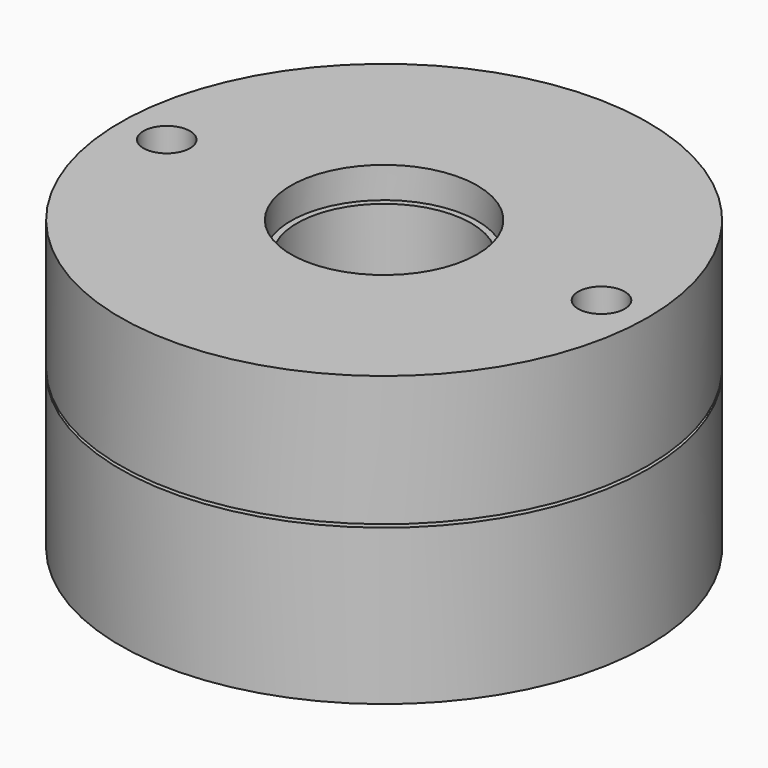
from build123d import *

# Parameters (mm, degrees)
F5_R      = 17
F5_W      = 21.2132034356
F5_H      = 21.2132034356
F5_R_2    = 8.1
F5_R_3    = 6
F6_DEPTH  = 0.5
F7_DEPTH  = 10
F9_DEPTH  = 0.9
F10_W     = 20.3646752982
F10_H     = 20.3646752982
F10_R     = 8.1
F11_DEPTH = 8.6
F12_R     = 1.1
F12_R_2   = 1
F14_W     = 2
F14_H     = 15
F18_R     = 17
F18_W     = 21.2132034356
F18_H     = 21.2132034356
F18_R_2   = 8.2
F18_R_3   = 6
F19_DEPTH = 2
F20_DEPTH = 6.4
F21_R     = 1.5
F22_DEPTH = 18.6


# Not quite as in the source:
# - a feature names something its author has since deleted; it is built from what else it names


with BuildPart() as f6:
    # F5 (on Top) → F6 (new body)
    with BuildSketch(Plane.XY):
        Circle(F5_R)
        with BuildLine():
            ThreePointArc((10.6066017178, 10.6066017178), (13.8581929877, 5.7402514855), (15, 0))
            ThreePointArc((15, 0), (13.8581929877, -5.7402514855), (10.6066017178, -10.6066017178))
            ThreePointArc((10.6066017178, -10.6066017178), (0, -15), (-10.6066017178, -10.6066017178))
            ThreePointArc((-10.6066017178, -10.6066017178), (-15, 0), (-10.6066017178, 10.6066017178))
            ThreePointArc((-10.6066017178, 10.6066017178), (0, 15), (10.6066017178, 10.6066017178))
        make_face(mode=Mode.SUBTRACT)
        with BuildLine():
            Line((-10.6066017178, 10.6066017178), (10.6066017178, 10.6066017178))
            ThreePointArc((10.6066017178, 10.6066017178), (0, 15), (-10.6066017178, 10.6066017178))
        make_face()
        with BuildLine():
            Line((-10.6066017178, -10.6066017178), (-10.6066017178, 10.6066017178))
            ThreePointArc((-10.6066017178, 10.6066017178), (-15, 0), (-10.6066017178, -10.6066017178))
        make_face()
        with BuildLine():
            ThreePointArc((10.6066017178, -10.6066017178), (13.8581929877, -5.7402514855), (15, 0))
            ThreePointArc((15, 0), (13.8581929877, 5.7402514855), (10.6066017178, 10.6066017178))
            Line((10.6066017178, 10.6066017178), (10.6066017178, -10.6066017178))
        make_face()
        with BuildLine():
            ThreePointArc((-10.6066017178, -10.6066017178), (0, -15), (10.6066017178, -10.6066017178))
            Line((10.6066017178, -10.6066017178), (-10.6066017178, -10.6066017178))
        make_face()
        Rectangle(F5_W, F5_H)
        Circle(F5_R_2, mode=Mode.SUBTRACT)
        Circle(F5_R_2)
        Circle(F5_R_3, mode=Mode.SUBTRACT)
    extrude(amount=F6_DEPTH)

    # F5 (on Top) → F7 (join)
    with BuildSketch(Plane.XY):
        Circle(F5_R)
        with BuildLine():
            ThreePointArc((10.6066017178, 10.6066017178), (13.8581929877, 5.7402514855), (15, 0))
            ThreePointArc((15, 0), (13.8581929877, -5.7402514855), (10.6066017178, -10.6066017178))
            ThreePointArc((10.6066017178, -10.6066017178), (0, -15), (-10.6066017178, -10.6066017178))
            ThreePointArc((-10.6066017178, -10.6066017178), (-15, 0), (-10.6066017178, 10.6066017178))
            ThreePointArc((-10.6066017178, 10.6066017178), (0, 15), (10.6066017178, 10.6066017178))
        make_face(mode=Mode.SUBTRACT)
        with BuildLine():
            Line((-10.6066017178, -10.6066017178), (-10.6066017178, 10.6066017178))
            ThreePointArc((-10.6066017178, 10.6066017178), (-15, 0), (-10.6066017178, -10.6066017178))
        make_face()
        with BuildLine():
            Line((-10.6066017178, 10.6066017178), (10.6066017178, 10.6066017178))
            ThreePointArc((10.6066017178, 10.6066017178), (0, 15), (-10.6066017178, 10.6066017178))
        make_face()
        with BuildLine():
            ThreePointArc((10.6066017178, -10.6066017178), (13.8581929877, -5.7402514855), (15, 0))
            ThreePointArc((15, 0), (13.8581929877, 5.7402514855), (10.6066017178, 10.6066017178))
            Line((10.6066017178, 10.6066017178), (10.6066017178, -10.6066017178))
        make_face()
        with BuildLine():
            ThreePointArc((-10.6066017178, -10.6066017178), (0, -15), (10.6066017178, -10.6066017178))
            Line((10.6066017178, -10.6066017178), (-10.6066017178, -10.6066017178))
        make_face()
    extrude(amount=F7_DEPTH)


with BuildPart() as f9:
    # F8 (on face) → F9 (new body)
    with BuildSketch(Plane.XY.offset(0.5)):
        with BuildLine():
            Line((10.3944696834, -10.3944696834), (10.3944696834, 10.3944696834))
            Line((10.3944696834, 10.3944696834), (-1.7686276827, 10.3944696834))
            Line((-1.7686276827, 10.3944696834), (-1.7686276827, 5.7334070255))
            ThreePointArc((-1.7686276827, 5.7334070255), (3.5628804291, 4.8276167048), (6, 0))
            ThreePointArc((6, 0), (3.5628804291, -4.8276167048), (-1.7686276827, -5.7334070255))
            Line((-1.7686276827, -5.7334070255), (-1.7686276827, -10.3944696834))
            Line((-1.7686276827, -10.3944696834), (10.3944696834, -10.3944696834))
        make_face()
    extrude(amount=F9_DEPTH)


with BuildPart() as f11:
    # F10 (on face) → F11 (new body)
    with BuildSketch(Plane.XY.offset(1.4)):
        Rectangle(F10_W, F10_H)
        Circle(F10_R, mode=Mode.SUBTRACT)
    extrude(amount=F11_DEPTH)

    # F12 (on Front) → F13 (revolve, cut)
    with BuildSketch(Plane.XZ):
        with Locations((8.5, 7.44)):
            Circle(F12_R)
        with Locations((8.5, 7.44)):
            Circle(F12_R_2, mode=Mode.SUBTRACT)
        with Locations((8.5, 4)):
            Circle(F12_R)
        with Locations((8.5, 4)):
            Circle(F12_R_2, mode=Mode.SUBTRACT)
        with Locations((8.5, 7.44)):
            Circle(F12_R_2)
        with Locations((8.5, 4)):
            Circle(F12_R_2)
    revolve(axis=Axis((0, 0, 11.7573533207), (0, 0, -1)), mode=Mode.SUBTRACT)


with BuildPart() as f15:
    # F14 (on Front) → F15 (revolve)
    with BuildSketch(Plane.XZ):
        with Locations((6.6, 9.1)):
            Rectangle(F14_W, F14_H)
    revolve(axis=Axis((0, 0, 5.7718302123), (0, 0, 1)))


with BuildPart() as f16:
    # F12 (on Front) → F16 (revolve)
    with BuildSketch(Plane.XZ):
        with Locations((8.5, 7.44)):
            Circle(F12_R_2)
    revolve(axis=Axis((0, 0, 11.7573533207), (0, 0, -1)))


with BuildPart() as f16b:
    # F12 (on Front) → F16, piece 2 (revolve)
    with BuildSketch(Plane.XZ):
        with Locations((8.5, 4)):
            Circle(F12_R_2)
    revolve(axis=Axis((0, 0, 11.7573533207), (0, 0, -1)))


with BuildPart() as f19:
    # F18 (on offset) → F19 (new body)
    with BuildSketch(Plane.XY.offset(16.6)):
        Circle(F18_R)
        with BuildLine():
            ThreePointArc((10.6066017178, 10.6066017178), (13.8581929877, 5.7402514855), (15, 0))
            ThreePointArc((15, 0), (13.8581929877, -5.7402514855), (10.6066017178, -10.6066017178))
            ThreePointArc((10.6066017178, -10.6066017178), (0, -15), (-10.6066017178, -10.6066017178))
            ThreePointArc((-10.6066017178, -10.6066017178), (-15, 0), (-10.6066017178, 10.6066017178))
            ThreePointArc((-10.6066017178, 10.6066017178), (0, 15), (10.6066017178, 10.6066017178))
        make_face(mode=Mode.SUBTRACT)
        Rectangle(F18_W, F18_H)
        Circle(F18_R_2, mode=Mode.SUBTRACT)
        Circle(F18_R_2)
        Circle(F18_R_3, mode=Mode.SUBTRACT)
        with BuildLine():
            Line((-10.6066017178, 10.6066017178), (10.6066017178, 10.6066017178))
            ThreePointArc((10.6066017178, 10.6066017178), (0, 15), (-10.6066017178, 10.6066017178))
        make_face()
        with BuildLine():
            Line((-10.6066017178, -10.6066017178), (-10.6066017178, 10.6066017178))
            ThreePointArc((-10.6066017178, 10.6066017178), (-15, 0), (-10.6066017178, -10.6066017178))
        make_face()
        with BuildLine():
            ThreePointArc((-10.6066017178, -10.6066017178), (0, -15), (10.6066017178, -10.6066017178))
            Line((10.6066017178, -10.6066017178), (-10.6066017178, -10.6066017178))
        make_face()
        with BuildLine():
            ThreePointArc((10.6066017178, -10.6066017178), (13.8581929877, -5.7402514855), (15, 0))
            ThreePointArc((15, 0), (13.8581929877, 5.7402514855), (10.6066017178, 10.6066017178))
            Line((10.6066017178, 10.6066017178), (10.6066017178, -10.6066017178))
        make_face()
    extrude(amount=F19_DEPTH)

    # F18 (on offset) → F20 (join)
    with BuildSketch(Plane.XY.offset(16.6)):
        Circle(F18_R)
        with BuildLine():
            ThreePointArc((10.6066017178, 10.6066017178), (13.8581929877, 5.7402514855), (15, 0))
            ThreePointArc((15, 0), (13.8581929877, -5.7402514855), (10.6066017178, -10.6066017178))
            ThreePointArc((10.6066017178, -10.6066017178), (0, -15), (-10.6066017178, -10.6066017178))
            ThreePointArc((-10.6066017178, -10.6066017178), (-15, 0), (-10.6066017178, 10.6066017178))
            ThreePointArc((-10.6066017178, 10.6066017178), (0, 15), (10.6066017178, 10.6066017178))
        make_face(mode=Mode.SUBTRACT)
        with BuildLine():
            ThreePointArc((-10.6066017178, -10.6066017178), (0, -15), (10.6066017178, -10.6066017178))
            Line((10.6066017178, -10.6066017178), (-10.6066017178, -10.6066017178))
        make_face()
        with BuildLine():
            Line((-10.6066017178, -10.6066017178), (-10.6066017178, 10.6066017178))
            ThreePointArc((-10.6066017178, 10.6066017178), (-15, 0), (-10.6066017178, -10.6066017178))
        make_face()
        with BuildLine():
            ThreePointArc((10.6066017178, -10.6066017178), (13.8581929877, -5.7402514855), (15, 0))
            ThreePointArc((15, 0), (13.8581929877, 5.7402514855), (10.6066017178, 10.6066017178))
            Line((10.6066017178, 10.6066017178), (10.6066017178, -10.6066017178))
        make_face()
        with BuildLine():
            Line((-10.6066017178, 10.6066017178), (10.6066017178, 10.6066017178))
            ThreePointArc((10.6066017178, 10.6066017178), (0, 15), (-10.6066017178, 10.6066017178))
        make_face()
    extrude(amount=-F20_DEPTH)


with BuildPart() as f22_tool:
    # F21 (on face) → F22 (new body, through all)
    with BuildSketch(Plane.XY.offset(18.6)):
        with Locations((-14, 0)):
            Circle(F21_R)
        with Locations((14, 0)):
            Circle(F21_R)
    extrude(amount=-F22_DEPTH)


with BuildPart() as f6_1:
    add(f6.part)

    # F22: cut by f22_tool
    add(f22_tool.part, mode=Mode.SUBTRACT)


with BuildPart() as f19_1:
    add(f19.part)

    # F22: cut by f22_tool
    add(f22_tool.part, mode=Mode.SUBTRACT)


solid = Compound([f9.part, f11.part, f15.part, f16.part, f16b.part, f6_1.part, f19_1.part])
